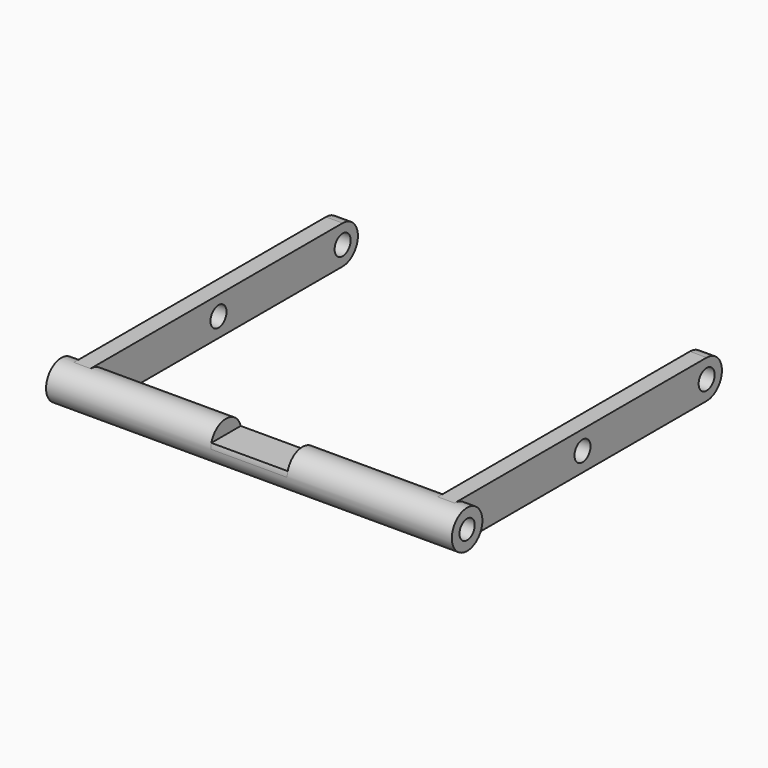
from build123d import *

# Parameters (mm, degrees)
F0_R          = 4
F1_DEPTH      = 42.5
F1_DEPTH_BACK = 42.5
F2_W          = 8
F2_H          = 8
F3_DEPTH      = 25
F4_W          = 3.5
F4_H          = 8
F5_DEPTH      = 70
F6_R          = 2
F7_DEPTH      = 25
F8_R          = 2
F9_DEPTH      = 25
F10_R         = 3.99999
F11_R         = 2.1
F12_DEPTH     = 82.3766380975
F14_DEPTH     = 16


# Not quite as in the source:
# - a fillet or chamfer is up to 0.001 mm smaller than in the source, because OpenCascade refuses the exact size


with BuildPart() as f1:
    # F0 (on Right) → F1 (new body, two sides)
    with BuildSketch(Plane.YZ) as f1_sk:
        Circle(F0_R)
    extrude(amount=F1_DEPTH)
    extrude(f1_sk.sketch, amount=-F1_DEPTH_BACK)

    # F2 (on Top) → F3 (cut)
    with BuildSketch(Plane.XY):
        with Locations((-4, 0)):
            Rectangle(F2_W, F2_H)
        with Locations((4, 0)):
            Rectangle(F2_W, F2_H)
    extrude(amount=F3_DEPTH, mode=Mode.SUBTRACT)

    # F4 (on Front) → F5 (join)
    with BuildSketch(Plane.XZ):
        with Locations((38.1256380975, 0)):
            Rectangle(F4_W, F4_H)
        with Locations((-38.1256380975, 0)):
            Rectangle(F4_W, F4_H)
    extrude(amount=-F5_DEPTH)

    # F6 (on face) → F7 (cut)
    with BuildSketch(Plane.YZ.offset(42.5)):
        Circle(F6_R)
    extrude(amount=-F7_DEPTH, mode=Mode.SUBTRACT)

    # F8 (on face) → F9 (cut)
    with BuildSketch(Plane(origin=(-42.5, 0, 0), x_dir=(0, -1, 0), z_dir=(-1, 0, 0))):
        Circle(F8_R)
    extrude(amount=-F9_DEPTH, mode=Mode.SUBTRACT)

    # F10 (radius 4 in the source; OpenCascade refuses exactly that, so slightly less here)
    f10_edges = [f1.edges().sort_by_distance(p)[0] for p in [
        (38.125638, 70, 4),
        (38.125638, 70, -4),
        (-38.125638, 70, 4),
        (-38.125638, 70, -4),
    ]]
    fillet(f10_edges, radius=F10_R)

    # F11 (on face) → F12 (cut, through all)
    with BuildSketch(Plane(origin=(-39.8756380975, 0, 0), x_dir=(0, -1, 0), z_dir=(-1, 0, 0))):
        with Locations((-66, 0)):
            Circle(F11_R)
        with Locations((-33.5, 0)):
            Circle(F11_R)
    extrude(amount=-F12_DEPTH, mode=Mode.SUBTRACT)

    # F13 (on face) → F14 (join, through all)
    with BuildSketch(Plane(origin=(8, 0, 0), x_dir=(0, -1, 0), z_dir=(-1, 0, 0))):
        with BuildLine():
            ThreePointArc((-3.848557921, 1.0902302184), (-3.9619585866, 0.5503491238), (-4, 0))
            Line((-4, 0), (4, 0))
            ThreePointArc((4, 0), (3.9619585866, 0.5503491238), (3.848557921, 1.0902302184))
            Line((3.848557921, 1.0902302184), (-3.848557921, 1.0902302184))
        make_face()
    extrude(amount=F14_DEPTH)


solid = f1.part
